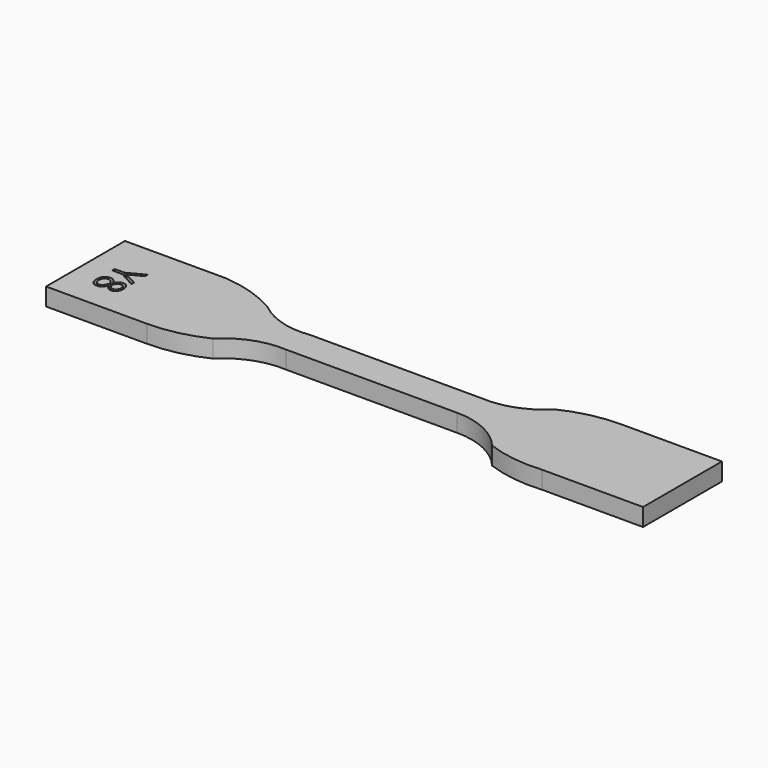
from build123d import *

# Parameters (mm, degrees)
F1_DEPTH     = 3.4
F2_TEXT_SIZE = 7.0564552314
F3_DEPTH     = 1


# Not quite as in the source:
# - Text() gives the source's letters only with a copy of the font that has no kerning and outlines rounded to 1/6400 em; it was checked with that copy


with BuildPart() as f1:
    # F0 (on Top) → F1 (new body)
    with BuildSketch(Plane.XY):
        with BuildLine():
            Line((-14.4320548165, 19.7811394548), (-33.8720548165, 19.7811394548))
            Line((-33.8720548165, 19.7811394548), (-33.8720548165, 0.7811394548))
            Line((-33.8720548165, 0.7811394548), (-14.4320548165, 0.7811394548))
            ThreePointArc((-14.4320548165, 0.7811394548), (-8.9053122052, 1.3996892086), (-3.6520548165, 3.2247301661))
            ThreePointArc((-3.6520548165, 3.2247301661), (1.3014698263, 6.4128780055), (7.1279451835, 7.2811394548))
            Line((7.1279451835, 7.2811394548), (40.1279451835, 7.2811394548))
            ThreePointArc((40.1279451835, 7.2811394548), (46.0837574042, 5.9511158081), (50.9079451835, 2.2137538538))
            ThreePointArc((50.9079451835, 2.2137538538), (56.2191047011, 0.9041953221), (61.6879451835, 0.7811394548))
            Line((61.6879451835, 0.7811394548), (81.1279451835, 0.7811394548))
            Line((81.1279451835, 0.7811394548), (81.1279451835, 19.7811394548))
            Line((81.1279451835, 19.7811394548), (61.6879451835, 19.7811394548))
            ThreePointArc((61.6879451835, 19.7811394548), (56.1612025723, 19.162589701), (50.9079451835, 17.3375487435))
            ThreePointArc((50.9079451835, 17.3375487435), (45.9544205407, 14.1494009041), (40.1279451835, 13.2811394548))
            Line((40.1279451835, 13.2811394548), (7.1279451835, 13.2811394548))
            ThreePointArc((7.1279451835, 13.2811394548), (1.4167452884, 13.6925537245), (-3.6520548165, 16.3560723447))
            ThreePointArc((-3.6520548165, 16.3560723447), (-8.8458057958, 18.686276846), (-14.4320548165, 19.7811394548))
        make_face()
    extrude(amount=F1_DEPTH)

    # F2 (on face) → F3 (cut)
    with BuildSketch(Plane.XY.offset(3.4)):
        with Locations(Location((-29.3720550835, 13.353464842), (0, 0, -90))):
            Text('Y8', F2_TEXT_SIZE, font='Open Sans', text_align=(TextAlign.LEFT, TextAlign.BOTTOM))
    extrude(amount=-F3_DEPTH, mode=Mode.SUBTRACT)


solid = f1.part
